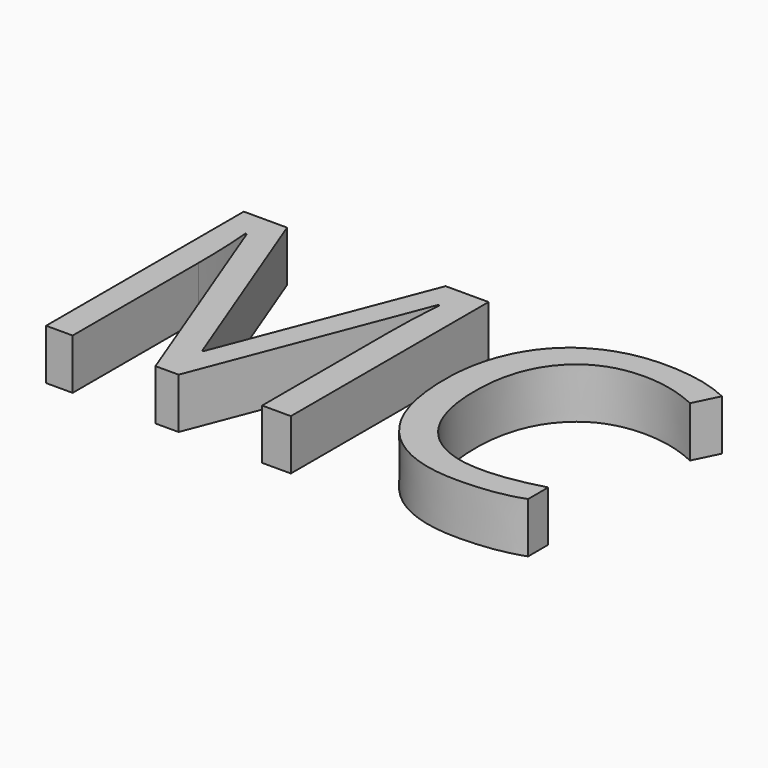
from build123d import *

# Parameters (mm, degrees)
F0_TEXT_SIZE = 6.8550932233
F1_DEPTH     = 1


# Not quite as in the source:
# - Text() gives the source's letters only with a copy of the font that has no kerning and outlines rounded to 1/6400 em; it was checked with that copy


with BuildPart() as f1:
    # F0 (on Top) → F1 (new body)
    with BuildSketch(Plane.XY):
        with Locations((-4.8645037604, -2.3954020638)):
            Text('MC', F0_TEXT_SIZE, font='Open Sans', text_align=(TextAlign.LEFT, TextAlign.BOTTOM))
    extrude(amount=F1_DEPTH)


solid = f1.part
